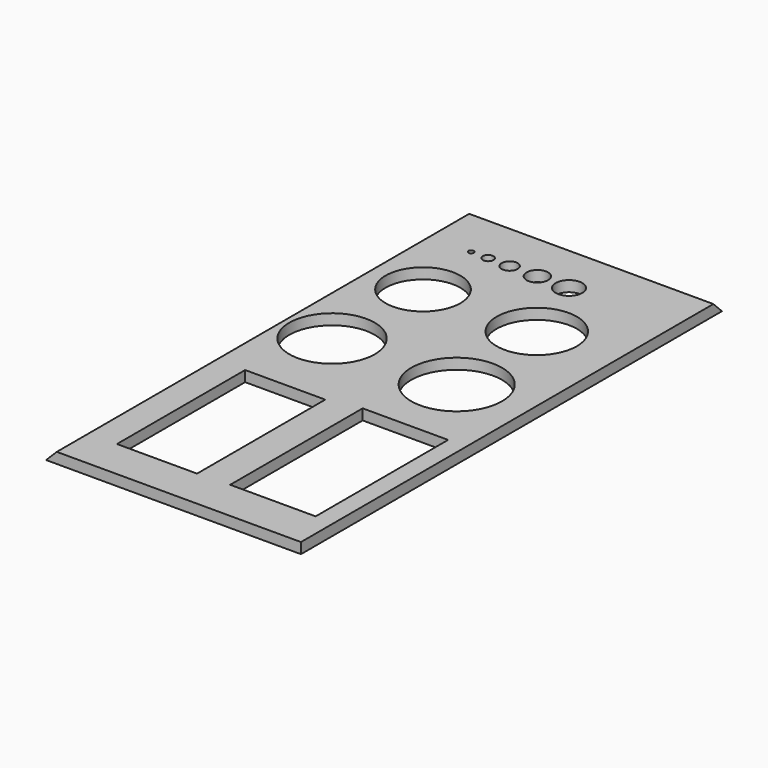
from build123d import *

# Parameters (mm, degrees)
F0_W        = 50.8
F0_H        = 101.6
F1_DEPTH    = 2
F2_T1_DEPTH = 127.7282991577
F2_T3_DEPTH = 76.9282991577
F3_W        = 15
F3_H        = 30
F3_W_2      = 16
F3_H_2      = 31
F3_R        = 8.5
F3_R_2      = 8
F3_R_3      = 7
F3_R_4      = 7.5
F3_R_5      = 2.5
F3_R_6      = 2
F3_R_7      = 1.5
F3_R_8      = 1
F3_R_9      = 0.5
F4_DEPTH    = 25.4


# Not quite as in the source:
# - a fillet or chamfer that OpenCascade refuses, or shapes differently, is made with other operations: its cross-section is extruded or revolved along the edge and cut away or added


with BuildPart() as f1:
    # F0 (on Top) → F1 (new body)
    with BuildSketch(Plane.XY):
        Rectangle(F0_W, F0_H)
    extrude(amount=F1_DEPTH)

    # F2: chamfer of 5.08 on 2 edges, made by hand

    # F2_s2 → F2_t1 (cut)
    with BuildSketch(Plane.XZ.offset(-63.8641495789)):
        Polygon((-25.4, -3.08), (-20.32, 2), (-25.4, 2), align=None)
    extrude(amount=F2_T1_DEPTH, mode=Mode.SUBTRACT)

    # F2_s4 → F2_t3 (cut)
    with BuildSketch(Plane.YZ.offset(-38.4641495789)):
        Polygon((50.8, -3.08), (45.72, 2), (50.8, 2), align=None)
    extrude(amount=F2_T3_DEPTH, mode=Mode.SUBTRACT)

    # F3 (on face) → F4 (cut)
    with BuildSketch(Plane.XY.offset(2)):
        with Locations((-7.5, -28.3660255373)):
            Rectangle(F3_W, F3_H)
        with Locations((13.9922183007, -27.6028160006)):
            Rectangle(F3_W_2, F3_H_2)
        with Locations((12.0123671368, 2.37495685)):
            Circle(F3_R)
        with Locations((-11.3166794181, 2.37495685)):
            Circle(F3_R_2)
        with Locations((-10.6418682262, 22.8119734675)):
            Circle(F3_R_3)
        with Locations((10.6627577916, 22.8119734675)):
            Circle(F3_R_4)
        with Locations((5.7463059202, 36.5009196103)):
            Circle(F3_R_5)
        with Locations((-0.1850809494, 36.5009196103)):
            Circle(F3_R_6)
        with Locations((-5.3699584678, 36.5009196103)):
            Circle(F3_R_7)
        with Locations((-9.3934237957, 36.5009196103)):
            Circle(F3_R_8)
        with Locations((-12.5698875636, 36.5009196103)):
            Circle(F3_R_9)
    extrude(amount=-F4_DEPTH, mode=Mode.SUBTRACT)


solid = f1.part
